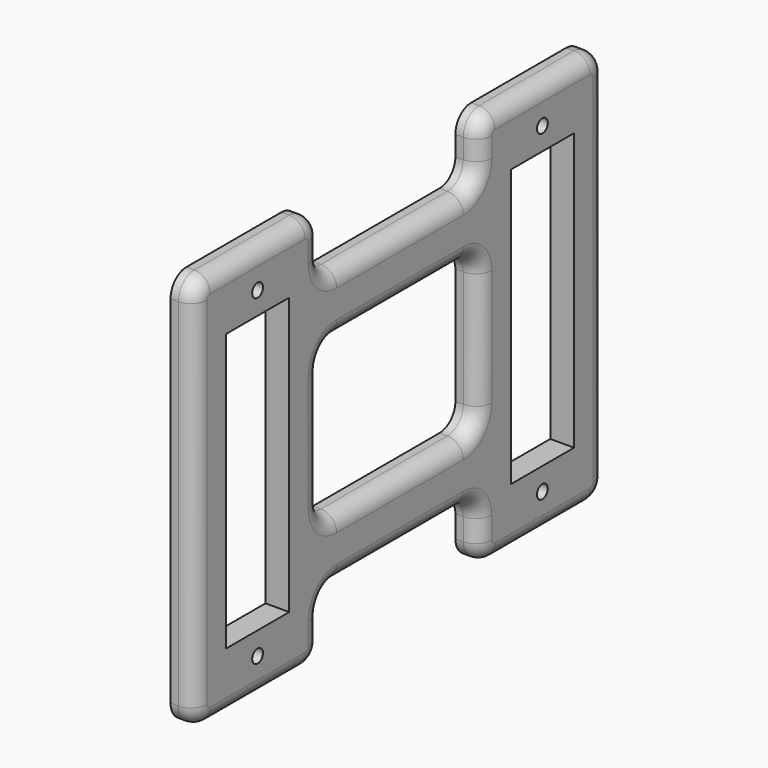
from build123d import *

# Parameters (mm, degrees)
F0_R        = 2.159
F0_W        = 25.4
F0_H        = 88.9
F1_DEPTH    = 7.62
F2_R        = 5.08
F3_T        = 3.81
F3_T3_DEPTH = 15.24


# Not quite as in the source:
# - a shell that OpenCascade refuses in one call is made with other operations: the cavity is built on its own and cut out


with BuildPart() as f1:
    # F0 (on Right) → F1 (new body)
    with BuildSketch(Plane.YZ):
        with BuildLine():
            Line((-36.5541661978, 94.9450524032), (-74.6541661978, 94.9450524032))
            ThreePointArc((-74.6541661978, 94.9450524032), (-79.1442942583, 93.0851804637), (-81.0041661978, 88.5950524032))
            Line((-81.0041661978, 88.5950524032), (-81.0041661978, -25.7049475968))
            ThreePointArc((-81.0041661978, -25.7049475968), (-79.1442942583, -30.1950756573), (-74.6541661978, -32.0549475968))
            Line((-74.6541661978, -32.0549475968), (-36.5541661978, -32.0549475968))
            ThreePointArc((-36.5541661978, -32.0549475968), (-32.0640381372, -30.1950756573), (-30.2041661978, -25.7049475968))
            Line((-30.2041661978, -25.7049475968), (-30.2041661978, -18.6545602813))
            ThreePointArc((-30.2041661978, -18.6545602813), (-28.3442942583, -14.1644322208), (-23.8541661978, -12.3045602813))
            Line((-23.8541661978, -12.3045602813), (26.9458338022, -12.3045602813))
            ThreePointArc((26.9458338022, -12.3045602813), (31.4359618628, -14.1644322208), (33.2958338022, -18.6545602813))
            Line((33.2958338022, -18.6545602813), (33.2958338022, -25.7049475968))
            ThreePointArc((33.2958338022, -25.7049475968), (35.1557057417, -30.1950756573), (39.6458338022, -32.0549475968))
            Line((39.6458338022, -32.0549475968), (77.7458338022, -32.0549475968))
            ThreePointArc((77.7458338022, -32.0549475968), (82.2359618628, -30.1950756573), (84.0958338022, -25.7049475968))
            Line((84.0958338022, -25.7049475968), (84.0958338022, 88.5950524032))
            ThreePointArc((84.0958338022, 88.5950524032), (82.2359618628, 93.0851804637), (77.7458338022, 94.9450524032))
            Line((77.7458338022, 94.9450524032), (39.6458338022, 94.9450524032))
            ThreePointArc((39.6458338022, 94.9450524032), (35.1557057417, 93.0851804637), (33.2958338022, 88.5950524032))
            Line((33.2958338022, 88.5950524032), (33.2958338022, 82.2450524032))
            ThreePointArc((33.2958338022, 82.2450524032), (31.4359618628, 77.7549243427), (26.9458338022, 75.8950524032))
            Line((26.9458338022, 75.8950524032), (-23.8541661978, 75.8950524032))
            ThreePointArc((-23.8541661978, 75.8950524032), (-28.3442942583, 77.7549243427), (-30.2041661978, 82.2450524032))
            Line((-30.2041661978, 82.2450524032), (-30.2041661978, 88.5950524032))
            ThreePointArc((-30.2041661978, 88.5950524032), (-32.0640381372, 93.0851804637), (-36.5541661978, 94.9450524032))
        make_face()
        with Locations((-55.6041661978, -20.2439475968)):
            Circle(F0_R, mode=Mode.SUBTRACT)
        with Locations((58.6958338022, -20.2439475968)):
            Circle(F0_R, mode=Mode.SUBTRACT)
        with Locations((-55.6041661978, 31.4450524032)):
            Rectangle(F0_W, F0_H, mode=Mode.SUBTRACT)
        with Locations((-55.6041661978, 83.1340524032)):
            Circle(F0_R, mode=Mode.SUBTRACT)
        with BuildLine():
            Line((26.9458338022, 6.7454397187), (-23.8541661978, 6.7454397187))
            ThreePointArc((-23.8541661978, 6.7454397187), (-28.3442942583, 8.6053116581), (-30.2041661978, 13.0954397187))
            Line((-30.2041661978, 13.0954397187), (-30.2041661978, 50.4950524032))
            ThreePointArc((-30.2041661978, 50.4950524032), (-28.3442942583, 54.9851804637), (-23.8541661978, 56.8450524032))
            Line((-23.8541661978, 56.8450524032), (26.9458338022, 56.8450524032))
            ThreePointArc((26.9458338022, 56.8450524032), (31.4359618628, 54.9851804637), (33.2958338022, 50.4950524032))
            Line((33.2958338022, 50.4950524032), (33.2958338022, 13.0954397187))
            ThreePointArc((33.2958338022, 13.0954397187), (31.4359618628, 8.6053116581), (26.9458338022, 6.7454397187))
        make_face(mode=Mode.SUBTRACT)
        with Locations((58.6958338022, 31.4450524032)):
            Rectangle(F0_W, F0_H, mode=Mode.SUBTRACT)
        with Locations((58.6958338022, 83.1340524032)):
            Circle(F0_R, mode=Mode.SUBTRACT)
    extrude(amount=F1_DEPTH)

    # F2
    f2_edges = [f1.edges().sort_by_distance(p)[0] for p in [
        (7.62, -55.604166, -32.054948),
        (7.62, 1.545834, 56.845052),
        (7.62, -55.604166, 94.945052),
        (7.62, -79.144294, 93.08518),
        (7.62, -81.004166, 31.445052),
        (7.62, -79.144294, -30.195076),
        (7.62, -32.064038, -30.195076),
        (7.62, -30.204166, -22.179754),
        (7.62, -28.344294, -14.164432),
        (7.62, 1.545834, -12.30456),
        (7.62, 31.435962, -14.164432),
        (7.62, 33.295834, -22.179754),
        (7.62, 35.155706, -30.195076),
        (7.62, 58.695834, -32.054948),
        (7.62, 82.235962, -30.195076),
        (7.62, 84.095834, 31.445052),
        (7.62, 82.235962, 93.08518),
        (7.62, 58.695834, 94.945052),
        (7.62, 35.155706, 93.08518),
        (7.62, 33.295834, 85.420052),
        (7.62, 31.435962, 77.754924),
        (7.62, 1.545834, 75.895052),
        (7.62, -28.344294, 77.754924),
        (7.62, -30.204166, 85.420052),
        (7.62, -32.064038, 93.08518),
        (7.62, 1.545834, 6.74544),
        (7.62, -28.344294, 8.605312),
        (7.62, -30.204166, 31.795246),
        (7.62, -28.344294, 54.98518),
        (7.62, 31.435962, 54.98518),
        (7.62, 33.295834, 31.795246),
        (7.62, 31.435962, 8.605312),
    ]]
    fillet(f2_edges, radius=F2_R)

    # F3: shell of thickness 3.81, made by hand


with BuildPart() as f3_core1:
    # F3_t2: copy of F1
    add(f1.part)

    # the walls: a layer under each face that stays
    f3_faces = [f3_core1.faces().sort_by_distance(p)[0] for p in [
        (1.27, -55.6041661978, 94.9450524032),
        (1.27, -32.0640381372, 93.0851804637),
        (6.1321024484, -55.6041661978, 93.4571548516),
        (1.27, -79.1442942583, 93.0851804637),
        (1.27, -30.2041661978, 85.4200524032),
        (6.1321024484, -33.1161405857, 92.0330780153),
        (7.62, 1.5458338022, 70.3917190699),
        (6.1321024484, -78.0921918099, 92.0330780153),
        (1.27, -81.0041661978, 31.4450524032),
        (1.27, -79.1442942583, -30.1950756573),
        (1.27, -55.6041661978, -32.0549475968),
        (1.27, -32.0640381372, -30.1950756573),
        (1.27, -30.2041661978, -22.1797539391),
        (1.27, -28.3442942583, -14.1644322208),
        (1.27, 1.5458338022, -12.3045602813),
        (1.27, 31.4359618628, -14.1644322208),
        (1.27, 33.2958338022, -22.1797539391),
        (1.27, 35.1557057417, -30.1950756573),
        (1.27, 58.6958338022, -32.0549475968),
        (1.27, 82.2359618628, -30.1950756573),
        (1.27, 84.0958338022, 31.4450524032),
        (1.27, 82.2359618628, 93.0851804637),
        (1.27, 58.6958338022, 94.9450524032),
        (1.27, 35.1557057417, 93.0851804637),
        (1.27, 33.2958338022, 85.4200524032),
        (1.27, 31.4359618628, 77.7549243427),
        (1.27, 1.5458338022, 75.8950524032),
        (1.27, -28.3442942583, 77.7549243427),
        (3.81, -57.7631661978, -20.2439475968),
        (3.81, 56.5368338022, -20.2439475968),
        (3.81, -42.9041661978, 31.4450524032),
        (3.81, -55.6041661978, -13.0049475968),
        (3.81, -68.3041661978, 31.4450524032),
        (3.81, -55.6041661978, 75.8950524032),
        (3.81, -57.7631661978, 83.1340524032),
        (1.27, 1.5458338022, 6.7454397187),
        (1.27, -28.3442942583, 8.6053116581),
        (1.27, -30.2041661978, 31.7952460609),
        (1.27, -28.3442942583, 54.9851804637),
        (1.27, 1.5458338022, 56.8450524032),
        (1.27, 31.4359618628, 54.9851804637),
        (1.27, 33.2958338022, 31.7952460609),
        (1.27, 31.4359618628, 8.6053116581),
        (3.81, 71.3958338022, 31.4450524032),
        (3.81, 58.6958338022, -13.0049475968),
        (3.81, 45.9958338022, 31.4450524032),
        (3.81, 58.6958338022, 75.8950524032),
        (3.81, 56.5368338022, 83.1340524032),
        (6.1321024484, -31.6920637493, 85.4200524032),
        (6.1321024484, -55.6041661978, -30.5670500452),
        (6.1321024484, -78.0921918099, -29.1429732089),
        (6.1321024484, -33.1161405857, -29.1429732089),
        (6.1321024484, -79.5162686462, 31.4450524032),
        (6.1321024484, -31.6920637493, -22.1797539391),
        (6.1321024484, -29.3963967067, -13.1123297724),
        (6.1321024484, 1.5458338022, -10.8166627298),
        (6.1321024484, 32.4880643112, -13.1123297724),
        (6.1321024484, 34.7837313538, -22.1797539391),
        (6.1321024484, -29.3963967067, 76.7028218942),
        (6.1321024484, 36.2078081901, -29.1429732089),
        (6.1321024484, 1.5458338022, 74.4071548516),
        (6.1321024484, 58.6958338022, -30.5670500452),
        (6.1321024484, 32.4880643112, 76.7028218942),
        (6.1321024484, 81.1838594143, -29.1429732089),
        (6.1321024484, 34.7837313538, 85.4200524032),
        (6.1321024484, 82.6079362507, 31.4450524032),
        (6.1321024484, 36.2078081901, 92.0330780153),
        (6.1321024484, 81.1838594143, 92.0330780153),
        (6.1321024484, 58.6958338022, 93.4571548516),
        (6.1321024484, 1.5458338022, 58.3329499548),
        (6.1321024484, -29.3963967067, 56.0372829122),
        (6.1321024484, 32.4880643112, 56.0372829122),
        (6.1321024484, -31.6920637493, 31.7952460609),
        (6.1321024484, 34.7837313538, 31.7952460609),
        (6.1321024484, -29.3963967067, 7.5532092097),
        (6.1321024484, 32.4880643112, 7.5532092097),
        (6.1321024484, 1.5458338022, 5.2575421671),
    ]]
    thicken(f3_faces, amount=-F3_T, mode=Mode.SUBTRACT)

    # F3_s4 → F3_t3 (cut)
    with BuildSketch(Plane.YZ.offset(-3.81)):
        Polygon((-42.9422661978, 75.8569524032), (-39.0941661978, 75.8950524032), (-39.0941661978, 79.7050524032), (-42.9041661978, 79.7050524032), align=None)
        Polygon((-42.9422661978, -12.9668475968), (-39.0941661978, -13.0049475968), (-39.0941661978, -16.8149475968), (-42.9041661978, -16.8149475968), align=None)
        Polygon((-68.2660661978, -12.9668475968), (-68.3041661978, -16.8149475968), (-72.1141661978, -16.8149475968), (-72.1141661978, -13.0049475968), align=None)
        Polygon((-68.2660661978, 75.8569524032), (-72.1141661978, 75.8950524032), (-72.1141661978, 79.7050524032), (-68.3041661978, 79.7050524032), align=None)
        Polygon((71.3577338022, 75.8569524032), (75.2058338022, 75.8950524032), (75.2058338022, 79.7050524032), (71.3958338022, 79.7050524032), align=None)
        Polygon((71.3577338022, -12.9668475968), (75.2058338022, -13.0049475968), (75.2058338022, -16.8149475968), (71.3958338022, -16.8149475968), align=None)
        Polygon((46.0339338022, -12.9668475968), (45.9958338022, -16.8149475968), (42.1858338022, -16.8149475968), (42.1858338022, -13.0049475968), align=None)
        Polygon((46.0339338022, 75.8569524032), (42.1858338022, 75.8950524032), (42.1858338022, 79.7050524032), (45.9958338022, 79.7050524032), align=None)
    extrude(amount=F3_T3_DEPTH, mode=Mode.SUBTRACT)


with BuildPart() as f1_1:
    add(f1.part)

    # what is left inside the walls is the cavity
    f3_cavity = [f3_core1.part.solids().sort_by_distance(p)[0] for p in [
        (0.0381, -37.824166, 51.341719),
    ]]
    add(f3_cavity, mode=Mode.SUBTRACT)


solid = f1_1.part
